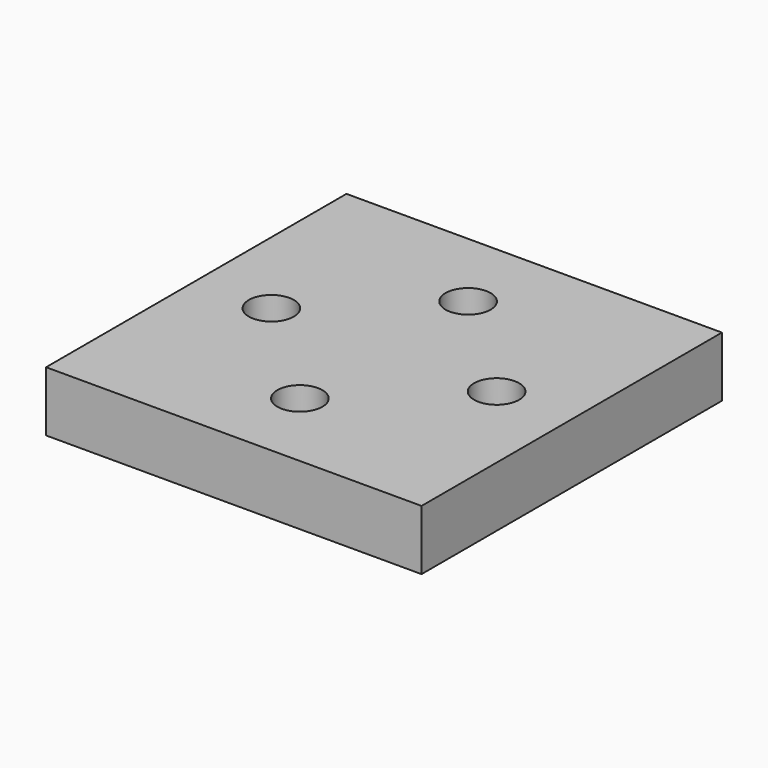
from build123d import *

# Parameters (mm, degrees)
F0_W     = 25
F0_H     = 25
F1_DEPTH = 4
F2_D     = 3


# Not quite as in the source:
# - a feature names something its author has since deleted; it is built from what else it names


with BuildPart() as f1:
    # F0 (on Top) → F1 (new body)
    with BuildSketch(Plane.XY):
        Rectangle(F0_W, F0_H)
    extrude(amount=F1_DEPTH)

    # F2 (through all)
    with Locations(Plane(origin=(0, 0, 0), x_dir=(1, 0, 0), z_dir=(0, 0, -1))):
        with Locations((-7.5, 0), (7.5, 0), (0, -7), (0, 7)):
            Hole(F2_D / 2)


solid = f1.part
